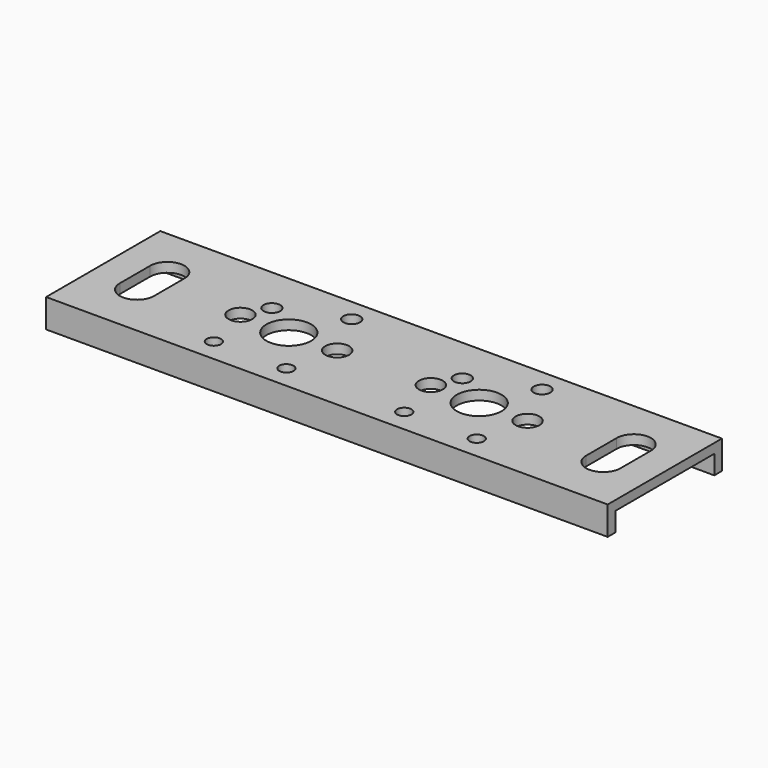
from build123d import *

# Parameters (mm, degrees)
F0_W        = 59
F0_H        = 15
F0_R        = 0.75
F0_R_2      = 1.25
F0_R_3      = 2.35
F0_R_4      = 0.875
F1_DEPTH    = 1
F2_W        = 0.5
F2_H        = 4
F3_DEPTH    = 3
F4_T4_DEPTH = 16.4300979278
F4_T9_DEPTH = 16.4300979278


# Not quite as in the source:
# - a fillet or chamfer that OpenCascade refuses, or shapes differently, is made with other operations: its cross-section is extruded or revolved along the edge and cut away or added


with BuildPart() as f1:
    # F0 (on Top) → F1 (new body)
    with BuildSketch(Plane.XY):
        with Locations((10, 12.3232733458)):
            Rectangle(F0_W, F0_H)
        with Locations((-3.81, 7.2432733458)):
            Circle(F0_R, mode=Mode.SUBTRACT)
        with Locations((3.81, 7.2432733458)):
            Circle(F0_R, mode=Mode.SUBTRACT)
        with Locations((-5.08, 12.3232733458)):
            Circle(F0_R_2, mode=Mode.SUBTRACT)
        with Locations((0, 12.3232733458)):
            Circle(F0_R_3, mode=Mode.SUBTRACT)
        with Locations((5.08, 12.3232733458)):
            Circle(F0_R_2, mode=Mode.SUBTRACT)
        with Locations((16.19, 7.2432733458)):
            Circle(F0_R, mode=Mode.SUBTRACT)
        with Locations((23.81, 7.2432733458)):
            Circle(F0_R, mode=Mode.SUBTRACT)
        with Locations((14.92, 12.3232733458)):
            Circle(F0_R_2, mode=Mode.SUBTRACT)
        with Locations((20, 12.3232733458)):
            Circle(F0_R_3, mode=Mode.SUBTRACT)
        with BuildLine():
            ThreePointArc((-16.3, 14.5025628582), (-14.5, 16.3025628582), (-12.7, 14.5025628582))
            Line((-12.7, 14.5025628582), (-12.7, 10.5025628582))
            ThreePointArc((-12.7, 10.5025628582), (-14.5, 8.7025628582), (-16.3, 10.5025628582))
            Line((-16.3, 10.5025628582), (-16.3, 14.5025628582))
        make_face(mode=Mode.SUBTRACT)
        with Locations((-3.81, 14.8632733458)):
            Circle(F0_R_4, mode=Mode.SUBTRACT)
        with Locations((2.54, 17.4032733458)):
            Circle(F0_R_4, mode=Mode.SUBTRACT)
        with Locations((16.19, 14.8632733458)):
            Circle(F0_R_4, mode=Mode.SUBTRACT)
        with Locations((25.08, 12.3232733458)):
            Circle(F0_R_2, mode=Mode.SUBTRACT)
        with BuildLine():
            ThreePointArc((36.3, 10.5025628582), (34.5, 8.7025628582), (32.7, 10.5025628582))
            Line((32.7, 10.5025628582), (32.7, 14.5025628582))
            ThreePointArc((32.7, 14.5025628582), (34.5, 16.3025628582), (36.3, 14.5025628582))
            Line((36.3, 14.5025628582), (36.3, 10.5025628582))
        make_face(mode=Mode.SUBTRACT)
        with Locations((22.54, 17.4032733458)):
            Circle(F0_R_4, mode=Mode.SUBTRACT)
    extrude(amount=F1_DEPTH)

    # F2 (on face) → F3 (join)
    with BuildSketch(Plane.XY.offset(1)):
        Polygon((39.5, 19.8232733458), (-19.5, 19.8232733458), (-19.5, 18.8232733458), (9.5, 18.8232733458), (10.5, 18.8232733458), (39.5, 18.8232733458), align=None)
        Polygon((9.5, 5.8232733458), (-19.5, 5.8232733458), (-19.5, 4.8232733458), (39.5, 4.8232733458), (39.5, 5.8232733458), (10.5, 5.8232733458), (10, 5.8232733458), align=None)
        with Locations((10.25, 7.8232733458)):
            Rectangle(F2_W, F2_H)
        Polygon((10.5, 18.8232733458), (9.5, 18.8232733458), (9.5, 14.8232733458), (10, 14.8232733458), (10.5, 14.8232733458), align=None)
        with Locations((9.75, 7.8232733458)):
            Rectangle(F2_W, F2_H)
    extrude(amount=-F3_DEPTH)

    # F4: chamfer of 3 on 2 edges, made by hand


with BuildPart() as f4_tool2:
    # F4_s3 → F4_t4 (new body)
    with BuildSketch(Plane.YZ.offset(18.2150489639)):
        Polygon((9.8232733458, 1), (6.8232733458, -2), (9.8232733458, -2), align=None)
    extrude(amount=-F4_T4_DEPTH)

    split(bisect_by=Plane.XY, keep=Keep.BOTTOM)


with BuildPart() as f1_1:
    add(f1.part)

    # F4_t1: cut F4_tool2
    add(f4_tool2.part, mode=Mode.SUBTRACT)


with BuildPart() as f4_tool7:
    # F4_s8 → F4_t9 (new body)
    with BuildSketch(Plane.YZ.offset(1.7849510361)):
        Polygon((14.8232733458, 1), (17.8232733458, -2), (14.8232733458, -2), align=None)
    extrude(amount=F4_T9_DEPTH)

    split(bisect_by=Plane.XY, keep=Keep.BOTTOM)


with BuildPart() as f1_2:
    add(f1_1.part)

    # F4_t6: cut F4_tool7
    add(f4_tool7.part, mode=Mode.SUBTRACT)


solid = f1_2.part
